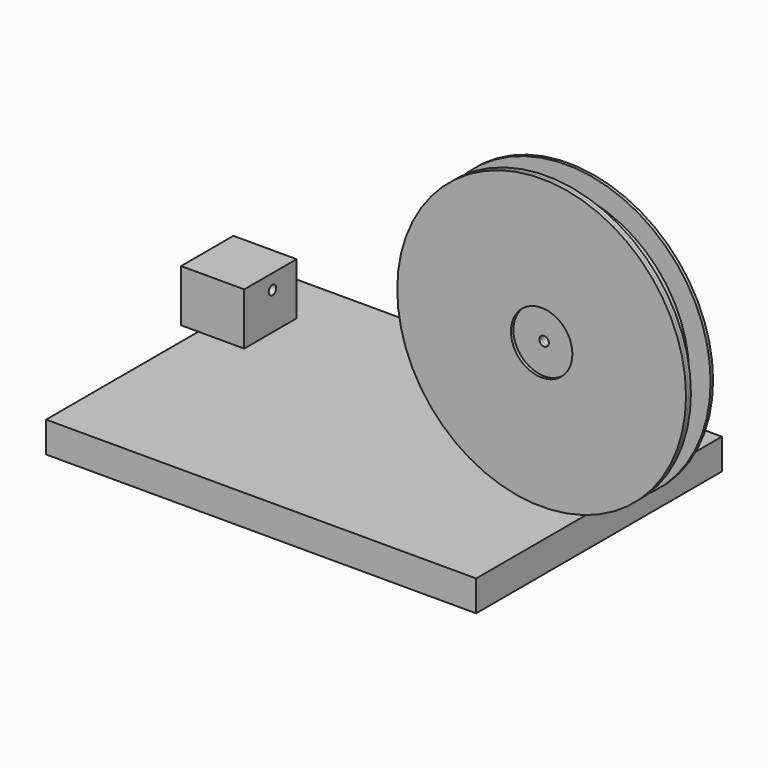
from build123d import *

# Parameters (mm, degrees)
F0_W           = 177.8
F0_H           = 127
F1_DEPTH       = 12.7
F2_W           = 26.1195935309
F2_H           = 21.5520188212
F3_DEPTH       = 27.05832
F4_R           = 1.9431
F5_DEPTH       = 9.46796
F6_R           = 50.8
F7_DEPTH       = 10.16
F6_R_2         = 59.69
F8_DEPTH       = 1.27
F9_R           = 1.9558
F10_DEPTH      = 25.4
F10_DEPTH_BACK = 75.06569
F9_R_2         = 59.69
F9_R_3         = 50.8
F9_R_4         = 12.7
F11_DEPTH      = 1.27
F11_FACE_R     = 59.69
F11_FACE_R_2   = 12.7
F12_DEPTH      = 1.27
F13_R          = 6.35
F14_DEPTH      = 25.4


# Not quite as in the source:
# - a length typed as a fraction of an inch, garbled in the dataset ("3 / 203.2 mm" for 3/8 in), is restored


with BuildPart() as f1:
    # F0 (on Top) → F1 (new body)
    with BuildSketch(Plane.XY):
        Rectangle(F0_W, F0_H)
    extrude(amount=F1_DEPTH)

    # F13 (on face) → F14 (cut)
    with BuildSketch(Plane.XY.offset(12.7)):
        with Locations((76.3196462645, 0)):
            Circle(F13_R)
    extrude(amount=-F14_DEPTH, mode=Mode.SUBTRACT)


with BuildPart() as f3:
    # F2 (on Front) → F3 (new body)
    with BuildSketch(Plane.XZ):
        with Locations((-49.19908382, 51.6582764685)):
            Rectangle(F2_W, F2_H)
    extrude(amount=F3_DEPTH)

    # F4 (on face) → F5 (cut)
    with BuildSketch(Plane.YZ.offset(-36.1392870545)):
        with Locations((-12.4484756961, 56.265860796)):
            Circle(F4_R)
    extrude(amount=-F5_DEPTH, mode=Mode.SUBTRACT)


with BuildPart() as f7:
    # F6 (on Front) → F7 (new body)
    with BuildSketch(Plane.XZ):
        with Locations((75.3328502178, 73.4556689858)):
            Circle(F6_R)
    extrude(amount=F7_DEPTH)

    # F6 (on Front) → F8 (join)
    with BuildSketch(Plane.XZ):
        with Locations((75.3328502178, 73.4556689858)):
            Circle(F6_R_2)
        with Locations((75.3328502178, 73.4556689858)):
            Circle(F6_R, mode=Mode.SUBTRACT)
        with Locations((75.3328502178, 73.4556689858)):
            Circle(F6_R)
    extrude(amount=-F8_DEPTH)

    # F9 (on face) → F10 (cut, two sides)
    with BuildSketch(Plane.XZ.offset(10.16)) as f10_sk:
        with Locations((75.3328502178, 73.4556689858)):
            Circle(F9_R)
    extrude(amount=-F10_DEPTH, mode=Mode.SUBTRACT)
    extrude(f10_sk.sketch, amount=F10_DEPTH_BACK, mode=Mode.SUBTRACT)

    # F9 (on face) → F11 (join)
    with BuildSketch(Plane.XZ.offset(10.16)):
        with Locations((75.3328502178, 73.4556689858)):
            Circle(F9_R_2)
        with Locations((75.3328502178, 73.4556689858)):
            Circle(F9_R_3, mode=Mode.SUBTRACT)
        with Locations((75.3328502178, 73.4556689858)):
            Circle(F9_R_3)
        with Locations((75.3328502178, 73.4556689858)):
            Circle(F9_R_4, mode=Mode.SUBTRACT)
    extrude(amount=F11_DEPTH)

    # F9 (on face) + F11_face (on face) → F12 (join)
    with BuildSketch(Plane.XZ.offset(10.16)):
        with Locations((75.3328502178, 73.4556689858)):
            Circle(F9_R_4)
        with Locations((75.3328502178, 73.4556689858)):
            Circle(F9_R, mode=Mode.SUBTRACT)
    with BuildSketch(Plane(origin=(75.3328502178, -11.43, 73.4556689858), x_dir=(1, 0, 0), z_dir=(0, -1, 0))):
        Circle(F11_FACE_R)
        Circle(F11_FACE_R_2, mode=Mode.SUBTRACT)
    extrude(amount=F12_DEPTH)


solid = Compound([f1.part, f3.part, f7.part])
